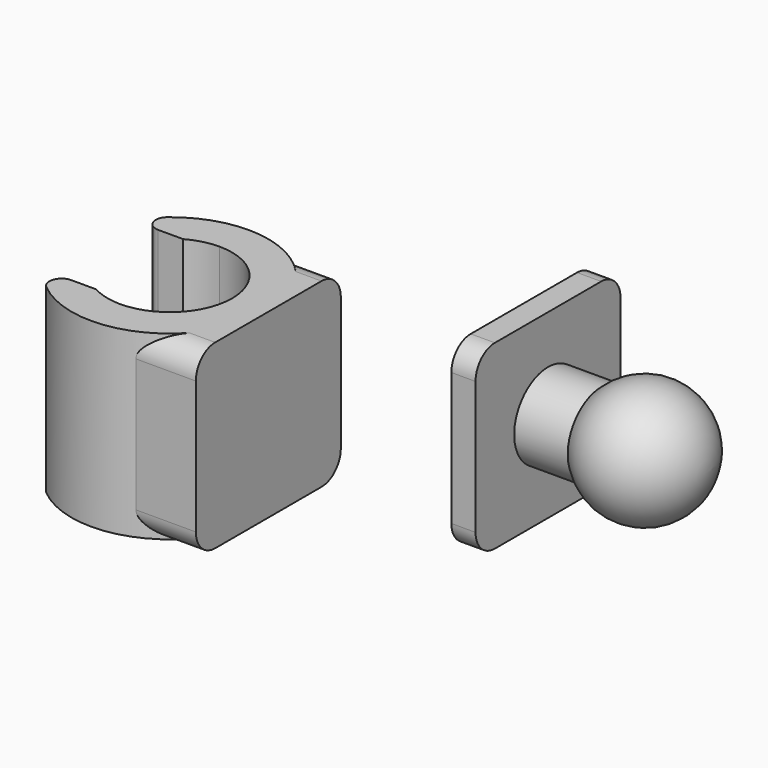
from build123d import *

# Parameters (mm, degrees)
F1_DEPTH = 15
F2_R     = 1
F6_DEPTH = 2
F7_R     = 2
F7_2_R   = 2


with BuildPart() as f1:
    # F0 (on Top) → F1 (new body)
    with BuildSketch(Plane.XY):
        with BuildLine():
            Line((-4.9605643132, 0), (0, 0))
            Line((0, 0), (0, 7.5))
            ThreePointArc((0, 7.5), (-1.3523386063, 3.0039684636), (-4.9605643132, 0))
        make_face()
        with BuildLine():
            ThreePointArc((-14.9450349521, 3), (-10.495226325, -0.3052811278), (-4.9605643132, 0))
            Line((-4.9605643132, 0), (-8.15, 0))
            Line((-8.15, 0), (-8.15, 2.35))
            ThreePointArc((-8.15, 2.35), (-9.4437349033, 2.515147946), (-10.6544959573, 3))
            Line((-10.6544959573, 3), (-14.9450349521, 3))
        make_face()
        with BuildLine():
            Line((-8.15, 0), (-4.9605643132, 0))
            ThreePointArc((-4.9605643132, 0), (-1.3523386063, 3.0039684636), (0, 7.5))
            ThreePointArc((0, 7.5), (-1.3523386063, 11.9960315364), (-4.9605643132, 15))
            Line((-4.9605643132, 15), (-8.15, 15))
            Line((-8.15, 15), (-8.15, 12.65))
            ThreePointArc((-8.15, 12.65), (-4.5084000769, 11.1415999231), (-3, 7.5))
            ThreePointArc((-3, 7.5), (-4.5084000769, 3.8584000769), (-8.15, 2.35))
            Line((-8.15, 2.35), (-8.15, 0))
        make_face()
        with BuildLine():
            ThreePointArc((-4.9605643132, 15), (-1.3523386063, 11.9960315364), (0, 7.5))
            Line((0, 7.5), (0, 15))
            Line((0, 15), (-4.9605643132, 15))
        make_face()
        with BuildLine():
            Line((-8.15, 15), (-4.9605643132, 15))
            ThreePointArc((-4.9605643132, 15), (-10.495226325, 15.3052811278), (-14.9450349521, 12))
            Line((-14.9450349521, 12), (-10.6544959573, 12))
            ThreePointArc((-10.6544959573, 12), (-9.4437349033, 12.484852054), (-8.15, 12.65))
            Line((-8.15, 12.65), (-8.15, 15))
        make_face()
    extrude(amount=F1_DEPTH)

    # F2
    f2_edges = [f1.edges().sort_by_distance(p)[0] for p in [
        (-14.945035, 12, 7.5),
        (-14.945035, 3, 7.5),
    ]]
    fillet(f2_edges, radius=F2_R)

    # F7
    f7_edges = [f1.edges().sort_by_distance(p)[0] for p in [
        (-2.480282, 0, 0),
        (-2.480282, 15, 0),
        (-2.480282, 15, 15),
        (-2.480282, 0, 15),
    ]]
    fillet(f7_edges, radius=F7_R)


with BuildPart() as f4:
    # F3 (on face) → F4 (revolve)
    with BuildSketch(Plane.XY.offset(15)):
        Polygon((21.1511792243, 15), (21.1511792243, 7.5), (23.1511792243, 7.5), (23.1511792243, 11), (23.1511792243, 15), align=None)
        with BuildLine():
            Line((23.1511792243, 11), (23.1511792243, 7.5))
            Line((23.1511792243, 7.5), (26.1511792243, 7.5))
            ThreePointArc((26.1511792243, 7.5), (26.5222716279, 9.3902948088), (27.58046501, 11))
            Line((27.58046501, 11), (23.1511792243, 11))
        make_face()
        with BuildLine():
            ThreePointArc((27.58046501, 11), (26.5222716279, 9.3902948088), (26.1511792243, 7.5))
            Line((26.1511792243, 7.5), (31.1511792243, 7.5))
            Line((31.1511792243, 7.5), (31.1511792243, 11))
            Line((31.1511792243, 11), (27.58046501, 11))
        make_face()
        with BuildLine():
            Line((31.1511792243, 7.5), (36.1511792243, 7.5))
            ThreePointArc((36.1511792243, 7.5), (33.0414740331, 12.1289075964), (27.58046501, 11))
            Line((27.58046501, 11), (31.1511792243, 11))
            Line((31.1511792243, 11), (31.1511792243, 7.5))
        make_face()
    revolve(axis=Axis((28.4954747185, 7.5, 15), (1, 0, 0)))

    # F5 (on face) → F6 (join)
    with BuildSketch(Plane(origin=(21.1511792243, 0, 0), x_dir=(0, -1, 0), z_dir=(-1, 0, 0))):
        with BuildLine():
            Line((-15, 15), (-15, 7.5))
            Line((-15, 7.5), (-7.5, 7.5))
            ThreePointArc((-7.5, 7.5), (-12.8033008589, 9.6966991411), (-15, 15))
        make_face()
        with BuildLine():
            Line((-15, 22.5), (-15, 15))
            ThreePointArc((-15, 15), (-12.8033008589, 20.3033008589), (-7.5, 22.5))
            Line((-7.5, 22.5), (-15, 22.5))
        make_face()
        with BuildLine():
            ThreePointArc((-7.5, 22.5), (-2.1966991411, 20.3033008589), (0, 15))
            Line((0, 15), (0, 22.5))
            Line((0, 22.5), (-7.5, 22.5))
        make_face()
        with BuildLine():
            ThreePointArc((0, 15), (-2.1966991411, 9.6966991411), (-7.5, 7.5))
            Line((-7.5, 7.5), (0, 7.5))
            Line((0, 7.5), (0, 15))
        make_face()
    extrude(amount=-F6_DEPTH)

    # F7#2
    f7_2_edges = [f4.edges().sort_by_distance(p)[0] for p in [
        (22.151179, 15, 22.5),
        (22.151179, 15, 7.5),
        (22.151179, 0, 7.5),
        (22.151179, 0, 22.5),
    ]]
    fillet(f7_2_edges, radius=F7_2_R)


solid = Compound([f1.part, f4.part])
